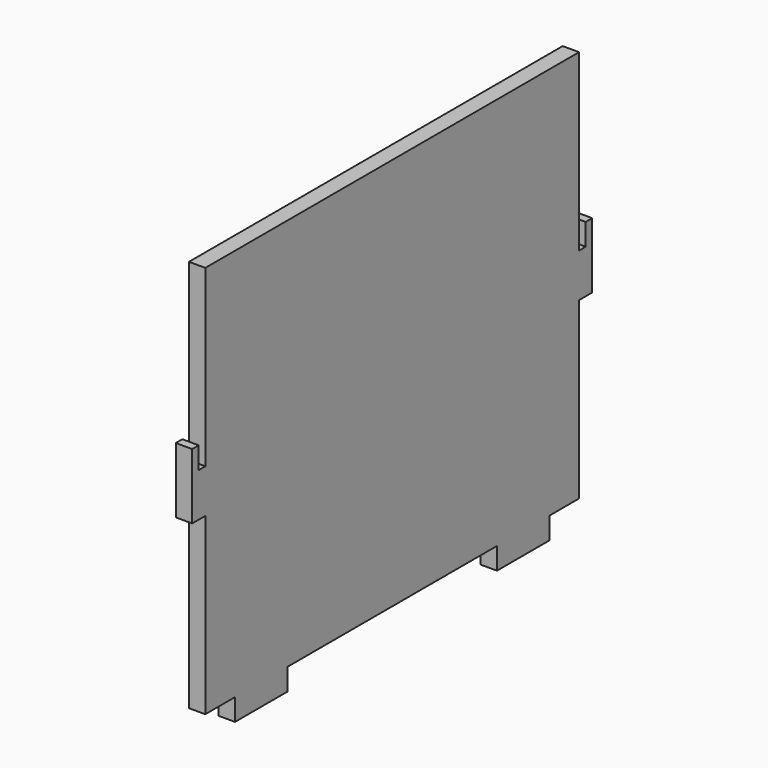
from build123d import *

# Parameters (mm, degrees)
F0_W      = 19.05
F0_H      = 543.56
F1_DEPTH  = 457.2
F2_W      = 19.05
F2_H      = 50.8
F3_DEPTH  = 19.1262
F4_W      = 19.05
F4_H      = 9.525
F5_DEPTH  = 25.4
F6_W      = 19.05
F6_H      = 50.8
F7_DEPTH  = 19.1262
F8_W      = 19.05
F8_H      = 9.525
F9_DEPTH  = 25.4
F10_W     = 19.05
F10_H     = 76.2
F11_DEPTH = 9.652
F12_DEPTH = 25.4


# Not quite as in the source:
# - a feature names something its author has since deleted; it is built from what else it names


with BuildPart() as f1:
    # F0 (on Top) → F1 (new body)
    with BuildSketch(Plane.XY):
        with Locations((-22.7488256648, 272.7919273724)):
            Rectangle(F0_W, F0_H)
    extrude(amount=F1_DEPTH)

    # F2 (on face) → F3 (join)
    with BuildSketch(Plane(origin=(0, 544.5719273724, 0), x_dir=(-1, 0, 0), z_dir=(0, 1, 0))):
        with Locations((22.7488256648, 228.6)):
            Rectangle(F2_W, F2_H)
    extrude(amount=F3_DEPTH)

    # F4 (on face) → F5 (join)
    with BuildSketch(Plane.XY.offset(254)):
        with Locations((-22.7488256648, 558.9356273724)):
            Rectangle(F4_W, F4_H)
    extrude(amount=F5_DEPTH)

    # F6 (on face) → F7 (join)
    with BuildSketch(Plane.XZ.offset(-1.0119273724)):
        with Locations((-22.7488256648, 228.6)):
            Rectangle(F6_W, F6_H)
    extrude(amount=F7_DEPTH)

    # F8 (on face) → F9 (join)
    with BuildSketch(Plane.XY.offset(254)):
        with Locations((-22.7488256648, -13.3517726276)):
            Rectangle(F8_W, F8_H)
    extrude(amount=F9_DEPTH)

    # F10 (on face) → F11 (join)
    with BuildSketch(Plane(origin=(0, 0, 0), x_dir=(1, 0, 0), z_dir=(0, 0, -1))):
        with Locations((-22.7488256648, -82.2919273724)):
            Rectangle(F10_W, F10_H)
        with Locations((-22.7488256648, -463.2919273724)):
            Rectangle(F10_W, F10_H)
    extrude(amount=F11_DEPTH)

    # F10 (on face) → F12 (join)
    with BuildSketch(Plane(origin=(0, 0, 0), x_dir=(1, 0, 0), z_dir=(0, 0, -1))):
        with Locations((-22.7488256648, -82.2919273724)):
            Rectangle(F10_W, F10_H)
        with Locations((-22.7488256648, -463.2919273724)):
            Rectangle(F10_W, F10_H)
    extrude(amount=F12_DEPTH)


solid = f1.part
